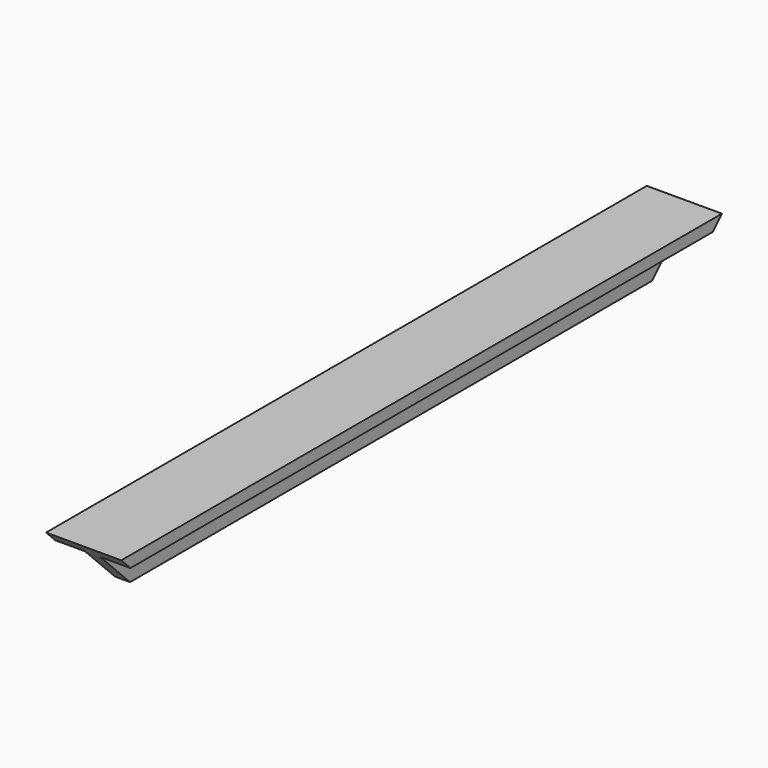
from build123d import *

# Parameters (mm, degrees)
F1_DEPTH    = 500
F2_T1_DEPTH = 359.4621544115
F3_T1_DEPTH = 359.4621544115


# Not quite as in the source:
# - a fillet or chamfer that OpenCascade refuses, or shapes differently, is made with other operations: its cross-section is extruded or revolved along the edge and cut away or added


with BuildPart() as f1:
    # F0 (on Front) → F1 (new body, symmetric)
    with BuildSketch(Plane.XZ):
        Polygon((50, -7.6415093219), (50, 7.6415093219), (-50, 7.6415093219), (-50, -7.6415093219), (-10.5660382013, -7.6415093219), (-1.1320764027, -7.6415093219), (0, -7.6415093219), (9.4339617987, -7.6415093219), align=None)
        Polygon((9.4339617987, -57.6415093219), (9.4339617987, -7.6415093219), (0, -7.6415093219), (-1.1320764027, -7.6415093219), (-10.5660382013, -7.6415093219), (-10.5660382013, -57.6415093219), align=None)
    extrude(amount=F1_DEPTH, both=True)

    # F2: chamfer of 66 on 1 edges, made by hand

    # F2_s2 → F2_t1 (cut)
    with BuildSketch(Plane.YZ.offset(-180.2971154071)):
        Polygon((434, -57.6415093219), (500, 8.3584906781), (500, -57.6415093219), align=None)
    extrude(amount=F2_T1_DEPTH, mode=Mode.SUBTRACT)

    # F3: chamfer of 66 on 1 edges, made by hand

    # F3_s2 → F3_t1 (cut)
    with BuildSketch(Plane.YZ.offset(-180.2971154071)):
        Polygon((-500, 8.3584906781), (-434, -57.6415093219), (-500, -57.6415093219), align=None)
    extrude(amount=F3_T1_DEPTH, mode=Mode.SUBTRACT)


solid = f1.part
